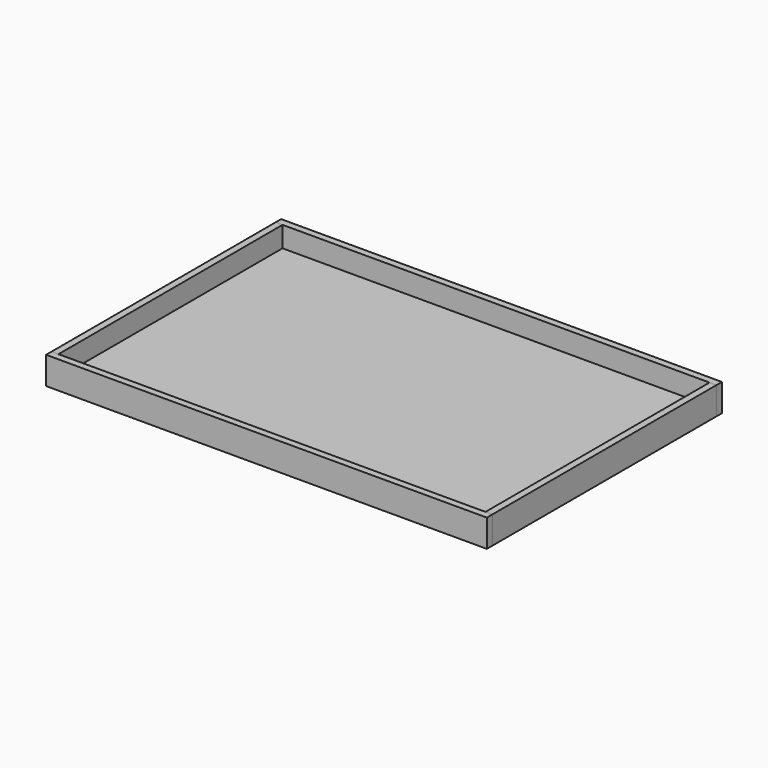
from build123d import *

# Parameters (mm, degrees)
F2_W     = 1181.1
F2_H     = 774.7
F3_DEPTH = 19.05
F5_DEPTH = 76.2
F7_W     = 19.05
F7_H     = 774.7
F8_DEPTH = 76.2


with BuildPart() as f3:
    # F2 (on Top) → F3 (new body, through all)
    with BuildSketch(Plane.XY):
        Rectangle(F2_W, F2_H)
    extrude(amount=F3_DEPTH)


with BuildPart() as f5:
    # F4 (on Top) → F5 (new body, through all)
    with BuildSketch(Plane.XY):
        Polygon((590.55, -387.35), (-590.55, -387.35), (-609.6, -387.35), (-609.6, -406.4), (609.6, -406.4), (609.6, -387.35), align=None)
    extrude(amount=F5_DEPTH)


with BuildPart() as f5b:
    # F4 (on Top) → F5, piece 2 (new body, through all)
    with BuildSketch(Plane.XY):
        Polygon((-609.6, 406.4), (-609.6, 387.35), (-590.55, 387.35), (590.55, 387.35), (609.6, 387.35), (609.6, 406.4), align=None)
    extrude(amount=F5_DEPTH)


with BuildPart() as f8:
    # F7 (on Top) → F8 (new body, through all)
    with BuildSketch(Plane.XY):
        with Locations((600.075, 0)):
            Rectangle(F7_W, F7_H)
    extrude(amount=F8_DEPTH)


with BuildPart() as f8b:
    # F7 (on Top) → F8, piece 2 (new body, through all)
    with BuildSketch(Plane.XY):
        with Locations((-600.075, 0)):
            Rectangle(F7_W, F7_H)
    extrude(amount=F8_DEPTH)


solid = Compound([f3.part, f5.part, f5b.part, f8.part, f8b.part])
